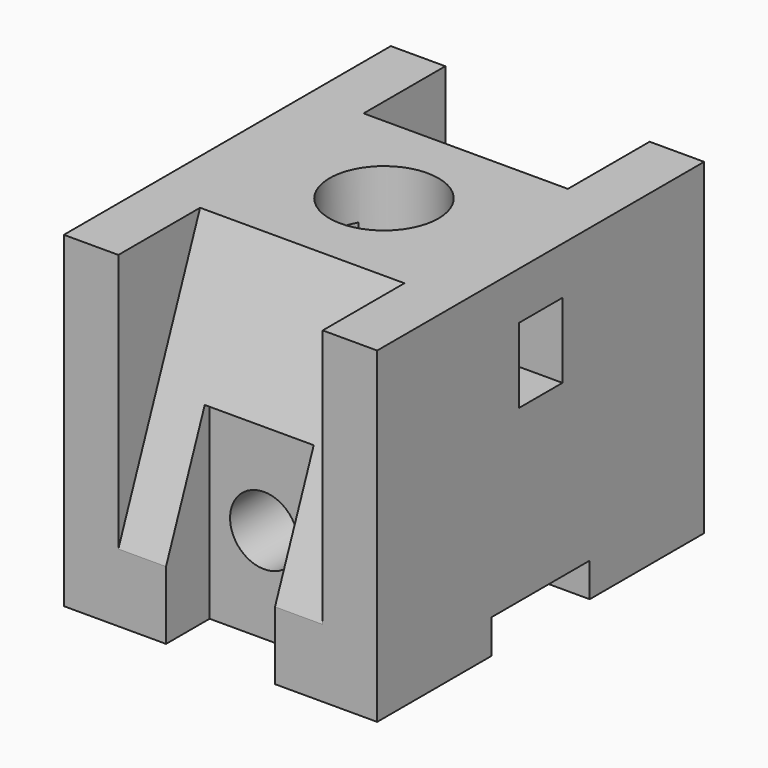
from build123d import *

# Parameters (mm, degrees)
F0_W      = 60
F0_H      = 48
F0_W_2    = 8
F0_H_2    = 11
F1_DEPTH  = 23
F2_W      = 18
F2_H      = 5
F3_DEPTH  = 46.001
F5_DEPTH  = 15
F6_R      = 8
F7_DEPTH  = 48.001
F8_W      = 16
F8_H      = 28
F9_DEPTH  = 8
F10_R     = 5
F11_DEPTH = 52.001


# Not quite as in the source:
# - a pattern or mirror of a feature is missing from the dataset's text; its kind, count and spacing are read off the source's solid


with BuildPart() as f1:
    # F0 (on Right) → F1 (new body, symmetric)
    with BuildSketch(Plane.YZ):
        Rectangle(F0_W, F0_H)
        with Locations((0, 11.5)):
            Rectangle(F0_W_2, F0_H_2, mode=Mode.SUBTRACT)
    extrude(amount=F1_DEPTH, both=True)

    # F2 (on face) → F3 (cut, through all)
    with BuildSketch(Plane.YZ.offset(23)):
        with Locations((0, -21.5)):
            Rectangle(F2_W, F2_H)
    extrude(amount=-F3_DEPTH, mode=Mode.SUBTRACT)

    # F4 (on Right) → F5 (cut, symmetric)
    with BuildSketch(Plane.YZ):
        Polygon((-15, 24), (-30, 24), (-30, -14), align=None)
    f5 = extrude(amount=F5_DEPTH, both=True, mode=Mode.SUBTRACT)

    # F5_copies: F5 across plane
    add(f5.mirror(Plane.ZX), mode=Mode.SUBTRACT)

    # F6 (on face) → F7 (cut, through all)
    with BuildSketch(Plane.XY.offset(24)):
        Circle(F6_R)
    extrude(amount=-F7_DEPTH, mode=Mode.SUBTRACT)

    # F8 (on face) → F9 (cut)
    with BuildSketch(Plane.XZ.offset(30)):
        with Locations((0, -10)):
            Rectangle(F8_W, F8_H)
    f9 = extrude(amount=-F9_DEPTH, mode=Mode.SUBTRACT)

    # F9_copies: F9 across plane
    add(f9.mirror(Plane.ZX), mode=Mode.SUBTRACT)

    # F10 (on face) → F11 (cut, through all)
    with BuildSketch(Plane.XZ.offset(22)):
        with Locations((0, -10)):
            Circle(F10_R)
    extrude(amount=-F11_DEPTH, mode=Mode.SUBTRACT)


solid = f1.part
